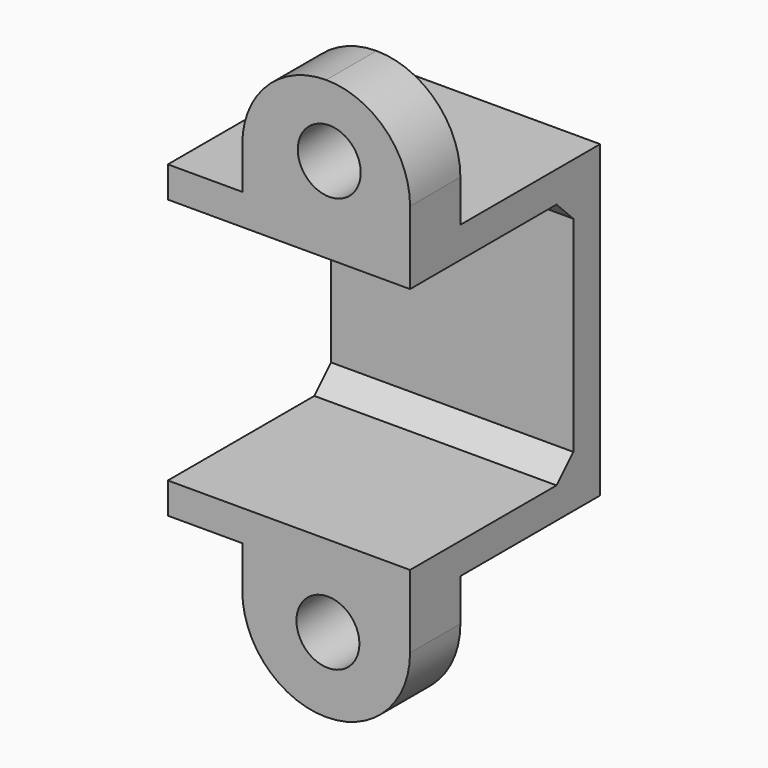
from build123d import *

# Parameters (mm, degrees)
F0_W      = 11.55
F0_H      = 1.48
F0_H_2    = 11.79
F1_DEPTH  = 11.33
F2_W      = 11.55
F2_H      = 11.79
F3_DEPTH  = 9.73
F4_W      = 3
F4_H      = 6
F5_DEPTH  = 8
F6_W      = 3
F6_H      = 6
F7_DEPTH  = 8
F8_R      = 4
F9_R      = 3.99999
F10_R     = 4
F11_R     = 3.99999
F12_R     = 1.5
F13_DEPTH = 25
F14_R     = 1.5
F15_DEPTH = 25
F16_SIZE  = 1
F17_SIZE  = 1


# Not quite as in the source:
# - a fillet or chamfer is up to 0.001 mm smaller than in the source, because OpenCascade refuses the exact size


with BuildPart() as f1:
    # F0 (on Front) → F1 (new body)
    with BuildSketch(Plane.XZ):
        with Locations((5.775, 0.74)):
            Rectangle(F0_W, F0_H)
        with Locations((5.775, 14.01)):
            Rectangle(F0_W, F0_H)
        with Locations((5.775, 7.375)):
            Rectangle(F0_W, F0_H_2)
    extrude(amount=F1_DEPTH)

    # F2 (on face) → F3 (cut)
    with BuildSketch(Plane.XZ.offset(11.33)):
        with Locations((5.775, 7.375)):
            Rectangle(F2_W, F2_H)
    extrude(amount=-F3_DEPTH, mode=Mode.SUBTRACT)

    # F4 (on face) → F5 (join)
    with BuildSketch(Plane.YZ.offset(11.55)):
        with Locations((-9.83, 17.75)):
            Rectangle(F4_W, F4_H)
        Polygon((-8.33, 14.75), (-11.33, 14.75), (-11.33, 13.27), (-1.6, 13.27), (-1.6, 1.48), (-11.33, 1.48), (-11.33, 0), (0, 0), (0, 14.75), align=None)
    extrude(amount=-F5_DEPTH)

    # F6 (on face) → F7 (join)
    with BuildSketch(Plane.YZ.offset(11.55)):
        with Locations((-9.83, -3)):
            Rectangle(F6_W, F6_H)
    extrude(amount=-F7_DEPTH)

    # F8
    f8_edges = [f1.edges().sort_by_distance(p)[0] for p in [
        (11.55, -9.83, 20.75),
    ]]
    fillet(f8_edges, radius=F8_R)

    # F9 (radius 4 in the source; OpenCascade refuses exactly that, so slightly less here)
    f9_edges = [f1.edges().sort_by_distance(p)[0] for p in [
        (3.55, -9.83, 20.75),
    ]]
    fillet(f9_edges, radius=F9_R)

    # F10
    f10_edges = [f1.edges().sort_by_distance(p)[0] for p in [
        (11.55, -9.83, -6),
    ]]
    fillet(f10_edges, radius=F10_R)

    # F11 (radius 4 in the source; OpenCascade refuses exactly that, so slightly less here)
    f11_edges = [f1.edges().sort_by_distance(p)[0] for p in [
        (3.55, -9.83, -6),
    ]]
    fillet(f11_edges, radius=F11_R)

    # F12 (on face) → F13 (cut)
    with BuildSketch(Plane(origin=(0, -8.33, 0), x_dir=(-1, 0, 0), z_dir=(0, 1, 0))):
        with Locations((-7.6327412389, -2.4092334788)):
            Circle(F12_R)
    extrude(amount=-F13_DEPTH, mode=Mode.SUBTRACT)

    # F14 (on face) → F15 (cut)
    with BuildSketch(Plane(origin=(0, -8.33, 0), x_dir=(-1, 0, 0), z_dir=(0, 1, 0))):
        with Locations((-7.6965787448, 17.3904672265)):
            Circle(F14_R)
    extrude(amount=-F15_DEPTH, mode=Mode.SUBTRACT)

    # F16
    f16_edges = [f1.edges().sort_by_distance(p)[0] for p in [
        (5.775, -1.6, 13.27),
    ]]
    chamfer(f16_edges, length=F16_SIZE)

    # F17
    f17_edges = [f1.edges().sort_by_distance(p)[0] for p in [
        (5.775, -1.6, 1.48),
    ]]
    chamfer(f17_edges, length=F17_SIZE)


solid = f1.part
